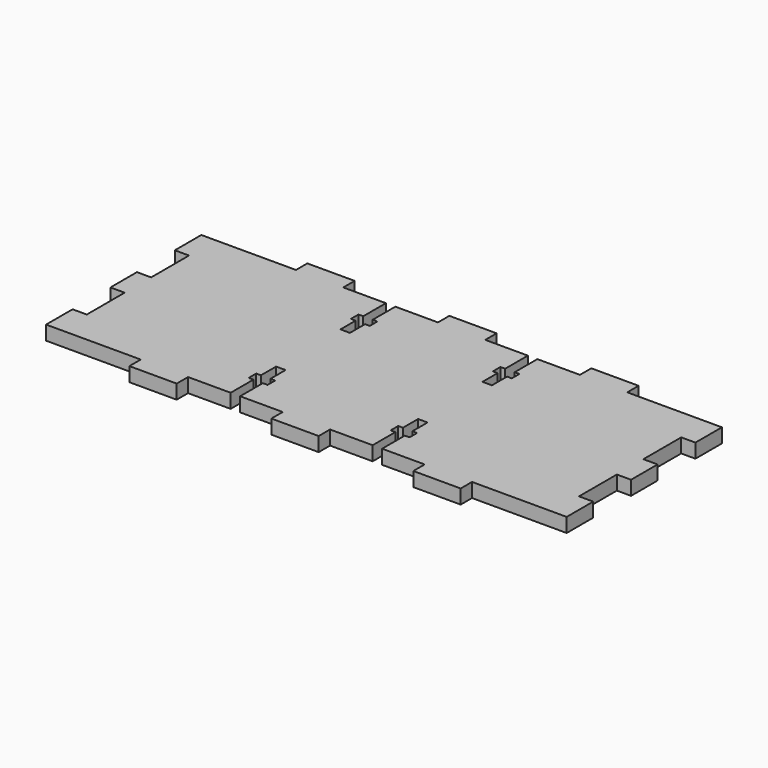
from build123d import *

# Parameters (mm, degrees)
F1_DEPTH = 3


# Not quite as in the source:
# - a feature names something its author has since deleted; it is built from what else it names


with BuildPart() as f1:
    # F0 (on Top) → F1 (new body)
    with BuildSketch(Plane.XY):
        Polygon((-7.6351782978, -15.3438961133), (2.3648217022, -15.3438961133), (2.3648217022, -12.3438961133), (11.3648217022, -12.3438961133), (11.3648217022, -6.3438961133), (10.3648217022, -6.3438961133), (10.3648217022, -4.3438961133), (11.3648217022, -4.3438961133), (11.3648217022, -0.3438961133), (13.3648217022, -0.3438961133), (13.3648217022, -4.3438961133), (14.3648217022, -4.3438961133), (14.3648217022, -6.3438961133), (13.3648217022, -6.3438961133), (13.3648217022, -12.3438961133), (22.3648217022, -12.3438961133), (22.3648217022, -15.3438961133), (32.3648217022, -15.3438961133), (32.3648217022, -12.3438961133), (52.3648217022, -12.3438961133), (52.3648217022, -5.3438961133), (49.3648217022, -5.3438961133), (49.3648217022, 4.6561038867), (52.3648217022, 4.6561038867), (52.3648217022, 11.6561038867), (49.3648217022, 11.6561038867), (49.3648217022, 21.6561038867), (52.3648217022, 21.6561038867), (52.3648217022, 28.6561038867), (32.3648217022, 28.6561038867), (32.3648217022, 31.6561038867), (22.3648217022, 31.6561038867), (22.3648217022, 28.6561038867), (13.3648217022, 28.6561038867), (13.3648217022, 22.6561038867), (14.3648217022, 22.6561038867), (14.3648217022, 20.6561038867), (13.3648217022, 20.6561038867), (13.3648217022, 16.6561038867), (11.3648217022, 16.6561038867), (11.3648217022, 20.6561038867), (10.3648217022, 20.6561038867), (10.3648217022, 22.6561038867), (11.3648217022, 22.6561038867), (11.3648217022, 28.6561038867), (2.3648217022, 28.6561038867), (2.3648217022, 31.6561038867), (-7.6351782978, 31.6561038867), (-7.6351782978, 28.6561038867), (-16.6351782978, 28.6561038867), (-16.6351782978, 22.6561038867), (-15.6351782978, 22.6561038867), (-15.6351782978, 20.6561038867), (-16.6351782978, 20.6561038867), (-16.6351782978, 16.6561038867), (-18.6351782978, 16.6561038867), (-18.6351782978, 20.6561038867), (-19.6351782978, 20.6561038867), (-19.6351782978, 22.6561038867), (-18.6351782978, 22.6561038867), (-18.6351782978, 28.6561038867), (-27.6351782978, 28.6561038867), (-27.6351782978, 31.6561038867), (-37.6351782978, 31.6561038867), (-37.6351782978, 28.6561038867), (-57.6351782978, 28.6561038867), (-57.6351782978, 21.6561038867), (-54.6351782978, 21.6561038867), (-54.6351782978, 11.6561038867), (-57.6351782978, 11.6561038867), (-57.6351782978, 4.6561038867), (-54.6351782978, 4.6561038867), (-54.6351782978, -5.3438961133), (-57.6351782978, -5.3438961133), (-57.6351782978, -12.3438961133), (-37.6351782978, -12.3438961133), (-37.6351782978, -15.3438961133), (-27.6351782978, -15.3438961133), (-27.6351782978, -12.3438961133), (-18.6351782978, -12.3438961133), (-18.6351782978, -6.3438961133), (-19.6351782978, -6.3438961133), (-19.6351782978, -4.3438961133), (-18.6351782978, -4.3438961133), (-18.6351782978, -0.3438961133), (-16.6351782978, -0.3438961133), (-16.6351782978, -4.3438961133), (-15.6351782978, -4.3438961133), (-15.6351782978, -6.3438961133), (-16.6351782978, -6.3438961133), (-16.6351782978, -12.3438961133), (-7.6351782978, -12.3438961133), align=None)
    extrude(amount=F1_DEPTH)


solid = f1.part
